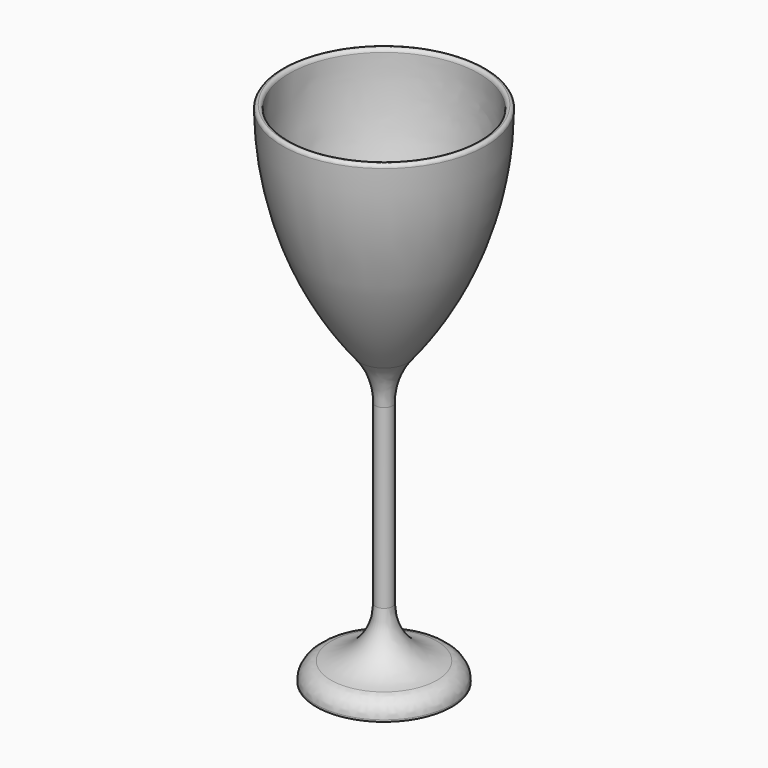
from build123d import *

# Parameters (mm, degrees)
F2_R = 15
F3_R = 5
F4_R = 20
F5_T = -2
F6_R = 0.999


# Not quite as in the source:
# - a fillet or chamfer is up to 0.001 mm smaller than in the source, because OpenCascade refuses the exact size


with BuildPart() as f1:
    # F0 (on Front) → F1 (revolve)
    with BuildSketch(Plane.XZ):
        with BuildLine():
            Line((30, 150), (0, 150))
            Line((0, 150), (0, 0))
            Line((0, 0), (20, 0))
            Line((20, 0), (20, 5))
            Line((20, 5), (2.5, 7))
            Line((2.5, 7), (2.5, 80))
            ThreePointArc((2.5, 80), (22.8784206322, 112.3959776088), (30, 150))
        make_face()
    revolve(axis=Axis((0, 0, 75), (0, 0, -1)))

    # F2
    f2_edges = [f1.edges().sort_by_distance(p)[0] for p in [
        (-2.5, 0, 7),
    ]]
    fillet(f2_edges, radius=F2_R)

    # F3
    f3_edges = [f1.edges().sort_by_distance(p)[0] for p in [
        (-20, 0, 5),
    ]]
    fillet(f3_edges, radius=F3_R)

    # F4
    f4_edges = [f1.edges().sort_by_distance(p)[0] for p in [
        (-2.5, 0, 80),
    ]]
    fillet(f4_edges, radius=F4_R)

    # F5
    f5_openings = [f1.faces().sort_by_distance(p)[0] for p in [
        (0, 0, 150),
    ]]
    offset(amount=F5_T, openings=f5_openings)

    # F6 (radius 1 in the source; OpenCascade refuses exactly that, so slightly less here)
    f6_edges = [f1.edges().sort_by_distance(p)[0] for p in [
        (-30, 0, 150),
        (-28, 0, 150),
    ]]
    fillet(f6_edges, radius=F6_R)


solid = f1.part
